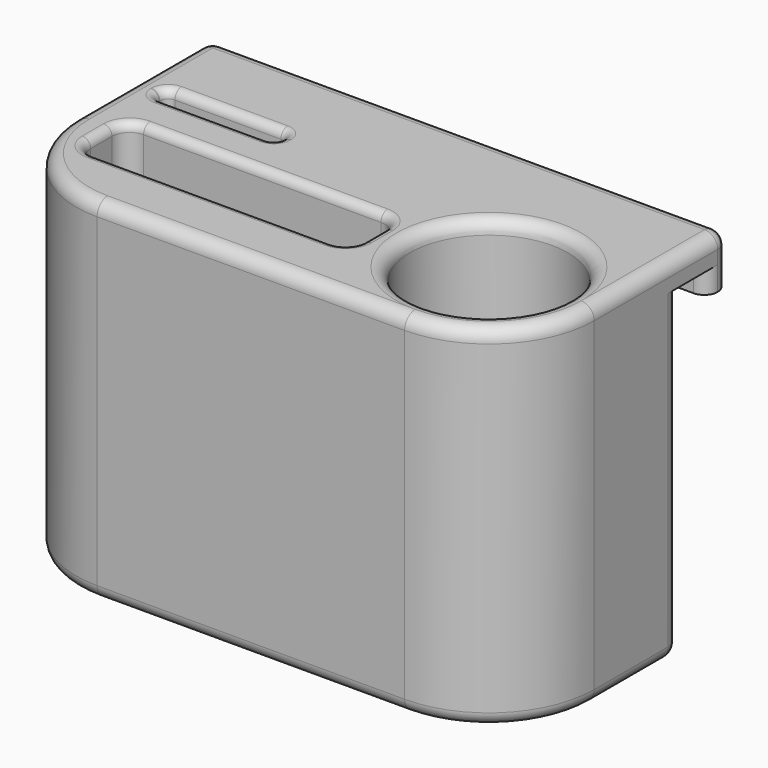
from build123d import *

# Parameters (mm, degrees)
F1_DEPTH     = 93.726
F3_DEPTH     = 63.5
F4_DEPTH     = 60.325
F6_DEPTH     = 63.501
F8_DEPTH     = 60.325
F9_T1_DEPTH  = 88.9508
F9_T3_DEPTH  = 27.9019
F9_T5_DEPTH  = 6.7564
F9_T7_DEPTH  = 56.2864
F9_T9_DEPTH  = 16.7259
F9_T11_DEPTH = 4.318
F9_T13_DEPTH = 55.626
F9_S17_W     = 2.435352
F9_S17_H     = 2.435352
F9_T18_DEPTH = 2.435352
F9_S23_W     = 2.435352
F9_S23_H     = 2.435352
F9_T24_DEPTH = 2.435352
F9_S29_W     = 2.435352
F9_S29_H     = 2.435352
F9_T30_DEPTH = 2.435352
F9_S35_W     = 2.435352
F9_S35_H     = 2.435352
F9_T36_DEPTH = 2.435352
F9_T42_ANGLE = 90
F9_T44_ANGLE = 90
F9_T46_ANGLE = 90
F9_T48_ANGLE = 90
F10_R        = 1.524


# Not quite as in the source:
# - a fillet or chamfer that OpenCascade refuses, or shapes differently, is made with other operations: its cross-section is extruded or revolved along the edge and cut away or added


with BuildPart() as f1:
    # F0 (on Right) → F1 (new body)
    with BuildSketch(Plane.YZ):
        Polygon((-6.35, 0), (0, 0), (0, -4.318), (4.826, -4.318), (4.826, 4.826), (-11.176, 4.826), (-11.176, -58.674), (-6.35, -58.674), align=None)
    extrude(amount=F1_DEPTH)

    # F2 (on face) → F3 (join, through all)
    with BuildSketch(Plane.XY.offset(4.826)):
        with BuildLine():
            Line((93.726, -11.176), (74.676, -11.176))
            Line((74.676, -11.176), (0, -11.176))
            Line((0, -11.176), (0, -25.4635))
            ThreePointArc((0, -25.4635), (5.5796158184, -38.9338841816), (19.05, -44.5135))
            Line((19.05, -44.5135), (74.676, -44.5135))
            ThreePointArc((74.676, -44.5135), (88.1463841816, -38.9338841816), (93.726, -25.4635))
            Line((93.726, -25.4635), (93.726, -11.176))
        make_face()
        with BuildLine():
            ThreePointArc((74.676, -11.176), (84.7787881362, -15.3607118638), (88.9635, -25.4635))
            ThreePointArc((88.9635, -25.4635), (64.5732118638, -35.5662881362), (74.676, -11.176))
        make_face(mode=Mode.SUBTRACT)
        with BuildLine():
            ThreePointArc((74.676, -11.176), (64.5732118638, -35.5662881362), (88.9635, -25.4635))
            ThreePointArc((88.9635, -25.4635), (84.7787881362, -15.3607118638), (74.676, -11.176))
        make_face()
    extrude(amount=-F3_DEPTH)

    # F2 (on face) → F4 (cut)
    with BuildSketch(Plane.XY.offset(4.826)):
        with BuildLine():
            ThreePointArc((74.676, -11.176), (64.5732118638, -35.5662881362), (88.9635, -25.4635))
            ThreePointArc((88.9635, -25.4635), (84.7787881362, -15.3607118638), (74.676, -11.176))
        make_face()
    extrude(amount=-F4_DEPTH, mode=Mode.SUBTRACT)

    # F5 (on face) → F6 (cut, through all)
    with BuildSketch(Plane.XY.offset(4.826)):
        with BuildLine():
            Line((25.527, -11.049), (6.35, -11.049))
            ThreePointArc((6.35, -11.049), (5.2723692655, -11.4953692655), (4.826, -12.573))
            Line((4.826, -12.573), (4.826, -12.7))
            ThreePointArc((4.826, -12.7), (5.2723692655, -13.7776307345), (6.35, -14.224))
            Line((6.35, -14.224), (25.527, -14.224))
            ThreePointArc((25.527, -14.224), (26.6046307345, -13.7776307345), (27.051, -12.7))
            Line((27.051, -12.7), (27.051, -12.573))
            ThreePointArc((27.051, -12.573), (26.6046307345, -11.4953692655), (25.527, -11.049))
        make_face()
    extrude(amount=-F6_DEPTH, mode=Mode.SUBTRACT)

    # F7 (on face) → F8 (cut, through all)
    with BuildSketch(Plane.XY.offset(4.826)):
        with BuildLine():
            ThreePointArc((55.626, -25.273), (54.6960640303, -23.0279359697), (52.451, -22.098))
            Line((52.451, -22.098), (9.525, -22.098))
            ThreePointArc((9.525, -22.098), (7.2799359697, -23.0279359697), (6.35, -25.273))
            Line((6.35, -25.273), (6.35, -30.099))
            ThreePointArc((6.35, -30.099), (7.2799359697, -32.3440640303), (9.525, -33.274))
            Line((9.525, -33.274), (52.451, -33.274))
            ThreePointArc((52.451, -33.274), (54.6960640303, -32.3440640303), (55.626, -30.099))
            Line((55.626, -30.099), (55.626, -25.273))
        make_face()
    extrude(amount=-F8_DEPTH, mode=Mode.SUBTRACT)

    # F9: fillet of radius 2.3876 on 11 edges, made by hand

    # F9_s2 → F9_t1 (cut)
    with BuildSketch(Plane.YZ.offset(2.3876)):
        with BuildLine():
            ThreePointArc((4.826, 2.4384), (4.1266881508, 4.1266881508), (2.4384, 4.826))
            Line((2.4384, 4.826), (2.4384, 4.873752))
            Line((2.4384, 4.873752), (4.873752, 4.873752))
            Line((4.873752, 4.873752), (4.873752, 2.4384))
            Line((4.873752, 2.4384), (4.826, 2.4384))
        make_face()
        with BuildLine():
            ThreePointArc((-8.7376, -58.674), (-7.0493118492, -57.9746881508), (-6.35, -56.2864))
            Line((-6.35, -56.2864), (-6.302248, -56.2864))
            Line((-6.302248, -56.2864), (-6.302248, -58.721752))
            Line((-6.302248, -58.721752), (-8.7376, -58.721752))
            Line((-8.7376, -58.721752), (-8.7376, -58.674))
        make_face()
    extrude(amount=F9_T1_DEPTH, mode=Mode.SUBTRACT)

    # F9_s4 → F9_t3 (cut)
    with BuildSketch(Plane.XZ.offset(-2.4384)):
        with BuildLine():
            ThreePointArc((0, 2.4384), (0.6993118492, 4.1266881508), (2.3876, 4.826))
            Line((2.3876, 4.826), (2.3876, 4.873752))
            Line((2.3876, 4.873752), (-0.047752, 4.873752))
            Line((-0.047752, 4.873752), (-0.047752, 2.4384))
            Line((-0.047752, 2.4384), (0, 2.4384))
        make_face()
        with BuildLine():
            ThreePointArc((93.726, 2.4384), (93.0266881508, 4.1266881508), (91.3384, 4.826))
            Line((91.3384, 4.826), (91.3384, 4.873752))
            Line((91.3384, 4.873752), (93.773752, 4.873752))
            Line((93.773752, 4.873752), (93.773752, 2.4384))
            Line((93.773752, 2.4384), (93.726, 2.4384))
        make_face()
    extrude(amount=F9_T3_DEPTH, mode=Mode.SUBTRACT)

    # F9_s6 → F9_t5 (cut)
    with BuildSketch(Plane.XY.offset(-4.318)):
        with BuildLine():
            ThreePointArc((0, 2.4384), (0.6993118492, 4.1266881508), (2.3876, 4.826))
            Line((2.3876, 4.826), (2.3876, 4.873752))
            Line((2.3876, 4.873752), (-0.047752, 4.873752))
            Line((-0.047752, 4.873752), (-0.047752, 2.4384))
            Line((-0.047752, 2.4384), (0, 2.4384))
        make_face()
        with BuildLine():
            ThreePointArc((93.726, 2.4384), (93.0266881508, 4.1266881508), (91.3384, 4.826))
            Line((91.3384, 4.826), (91.3384, 4.873752))
            Line((91.3384, 4.873752), (93.773752, 4.873752))
            Line((93.773752, 4.873752), (93.773752, 2.4384))
            Line((93.773752, 2.4384), (93.726, 2.4384))
        make_face()
    extrude(amount=F9_T5_DEPTH, mode=Mode.SUBTRACT)

    # F9_s8 → F9_t7 (cut)
    with BuildSketch(Plane.XY.offset(-56.2864)):
        with BuildLine():
            ThreePointArc((2.3876, -6.35), (0.6993118492, -7.0493118492), (0, -8.7376))
            Line((0, -8.7376), (-0.047752, -8.7376))
            Line((-0.047752, -8.7376), (-0.047752, -6.302248))
            Line((-0.047752, -6.302248), (2.3876, -6.302248))
            Line((2.3876, -6.302248), (2.3876, -6.35))
        make_face()
        with BuildLine():
            ThreePointArc((91.3384, -6.35), (93.0266881508, -7.0493118492), (93.726, -8.7376))
            Line((93.726, -8.7376), (93.773752, -8.7376))
            Line((93.773752, -8.7376), (93.773752, -6.302248))
            Line((93.773752, -6.302248), (91.3384, -6.302248))
            Line((91.3384, -6.302248), (91.3384, -6.35))
        make_face()
    extrude(amount=F9_T7_DEPTH, mode=Mode.SUBTRACT)

    # F9_s10 → F9_t9 (cut)
    with BuildSketch(Plane.XZ.offset(8.7376)):
        with BuildLine():
            ThreePointArc((2.3876, -58.674), (0.6993118492, -57.9746881508), (0, -56.2864))
            Line((0, -56.2864), (-0.047752, -56.2864))
            Line((-0.047752, -56.2864), (-0.047752, -58.721752))
            Line((-0.047752, -58.721752), (2.3876, -58.721752))
            Line((2.3876, -58.721752), (2.3876, -58.674))
        make_face()
        with BuildLine():
            ThreePointArc((91.3384, -58.674), (93.0266881508, -57.9746881508), (93.726, -56.2864))
            Line((93.726, -56.2864), (93.773752, -56.2864))
            Line((93.773752, -56.2864), (93.773752, -58.721752))
            Line((93.773752, -58.721752), (91.3384, -58.721752))
            Line((91.3384, -58.721752), (91.3384, -58.674))
        make_face()
    extrude(amount=F9_T9_DEPTH, mode=Mode.SUBTRACT)

    # F9_s12 → F9_t11 (cut)
    with BuildSketch(Plane.XY.offset(-4.318)):
        with BuildLine():
            ThreePointArc((0, 2.3876), (0.6993118492, 0.6993118492), (2.3876, 0))
            Line((2.3876, 0), (2.3876, -0.047752))
            Line((2.3876, -0.047752), (-0.047752, -0.047752))
            Line((-0.047752, -0.047752), (-0.047752, 2.3876))
            Line((-0.047752, 2.3876), (0, 2.3876))
        make_face()
        with BuildLine():
            ThreePointArc((93.726, 2.3876), (93.0266881508, 0.6993118492), (91.3384, 0))
            Line((91.3384, 0), (91.3384, -0.047752))
            Line((91.3384, -0.047752), (93.773752, -0.047752))
            Line((93.773752, -0.047752), (93.773752, 2.3876))
            Line((93.773752, 2.3876), (93.726, 2.3876))
        make_face()
    extrude(amount=F9_T11_DEPTH, mode=Mode.SUBTRACT)

    # F9_s14 → F9_t13 (cut)
    with BuildSketch(Plane.YZ.offset(19.05)):
        with BuildLine():
            ThreePointArc((-42.1259, -58.674), (-43.8141881508, -57.9746881508), (-44.5135, -56.2864))
            Line((-44.5135, -56.2864), (-44.561252, -56.2864))
            Line((-44.561252, -56.2864), (-44.561252, -58.721752))
            Line((-44.561252, -58.721752), (-42.1259, -58.721752))
            Line((-42.1259, -58.721752), (-42.1259, -58.674))
        make_face()
        with BuildLine():
            ThreePointArc((-44.5135, 2.4384), (-43.8141881508, 4.1266881508), (-42.1259, 4.826))
            Line((-42.1259, 4.826), (-42.1259, 4.873752))
            Line((-42.1259, 4.873752), (-44.561252, 4.873752))
            Line((-44.561252, 4.873752), (-44.561252, 2.4384))
            Line((-44.561252, 2.4384), (-44.5135, 2.4384))
        make_face()
    extrude(amount=F9_T13_DEPTH, mode=Mode.SUBTRACT)


with BuildPart() as f9_tool16:
    # F9_s17 → F9_t18 (new body)
    with BuildSketch(Plane.YZ.offset(2.3876)):
        with Locations((3.656076, 3.656076)):
            Rectangle(F9_S17_W, F9_S17_H)
    extrude(amount=-F9_T18_DEPTH)

    # F9_s19 → F9_t20 (revolve, cut)
    with BuildSketch(Plane(origin=(2.3876, 2.4384, 2.4384), x_dir=(0, -0.7071067812, -0.7071067812), z_dir=(0, 0.7071067812, -0.7071067812))):
        with BuildLine():
            ThreePointArc((0, -2.3876), (2.3876, 0), (0, 2.3876))
            Line((0, 2.3876), (0, -2.3876))
        make_face()
    revolve(axis=Axis((2.3876, 2.4384, 2.4384), (-1, 0, 0)), mode=Mode.SUBTRACT)


with BuildPart() as f1_1:
    add(f1.part)

    # F9_t15: cut F9_tool16
    add(f9_tool16.part, mode=Mode.SUBTRACT)


with BuildPart() as f9_tool22:
    # F9_s23 → F9_t24 (new body)
    with BuildSketch(Plane.YZ.offset(91.3384)):
        with Locations((3.656076, 3.656076)):
            Rectangle(F9_S23_W, F9_S23_H)
    extrude(amount=F9_T24_DEPTH)

    # F9_s25 → F9_t26 (revolve, cut)
    with BuildSketch(Plane(origin=(91.3384, 2.4384, 2.4384), x_dir=(0, -0.7071067812, -0.7071067812), z_dir=(0, -0.7071067812, 0.7071067812))):
        with BuildLine():
            ThreePointArc((0, -2.3876), (2.3876, 0), (0, 2.3876))
            Line((0, 2.3876), (0, -2.3876))
        make_face()
    revolve(axis=Axis((91.3384, 2.4384, 2.4384), (1, 0, 0)), mode=Mode.SUBTRACT)


with BuildPart() as f1_2:
    add(f1_1.part)

    # F9_t21: cut F9_tool22
    add(f9_tool22.part, mode=Mode.SUBTRACT)


with BuildPart() as f9_tool28:
    # F9_s29 → F9_t30 (new body)
    with BuildSketch(Plane.XY.offset(-56.2864)):
        with Locations((1.169924, -7.519924)):
            Rectangle(F9_S29_W, F9_S29_H)
    extrude(amount=-F9_T30_DEPTH)

    # F9_s31 → F9_t32 (revolve, cut)
    with BuildSketch(Plane(origin=(2.3876, -8.7376, -56.2864), x_dir=(0.7071067812, -0.7071067812, 0), z_dir=(0.7071067812, 0.7071067812, 0))):
        with BuildLine():
            ThreePointArc((0, -2.3876), (2.3876, 0), (0, 2.3876))
            Line((0, 2.3876), (0, -2.3876))
        make_face()
    revolve(axis=Axis((2.3876, -8.7376, -56.2864), (0, 0, -1)), mode=Mode.SUBTRACT)


with BuildPart() as f1_3:
    add(f1_2.part)

    # F9_t27: cut F9_tool28
    add(f9_tool28.part, mode=Mode.SUBTRACT)


with BuildPart() as f9_tool34:
    # F9_s35 → F9_t36 (new body)
    with BuildSketch(Plane.XY.offset(-56.2864)):
        with Locations((92.556076, -7.519924)):
            Rectangle(F9_S35_W, F9_S35_H)
    extrude(amount=-F9_T36_DEPTH)

    # F9_s37 → F9_t38 (revolve, cut)
    with BuildSketch(Plane(origin=(91.3384, -8.7376, -56.2864), x_dir=(-0.7071067812, -0.7071067812, 0), z_dir=(0.7071067812, -0.7071067812, 0))):
        with BuildLine():
            ThreePointArc((0, -2.3876), (2.3876, 0), (0, 2.3876))
            Line((0, 2.3876), (0, -2.3876))
        make_face()
    revolve(axis=Axis((91.3384, -8.7376, -56.2864), (0, 0, -1)), mode=Mode.SUBTRACT)


with BuildPart() as f1_4:
    add(f1_3.part)

    # F9_t33: cut F9_tool34
    add(f9_tool34.part, mode=Mode.SUBTRACT)

    # F9_s39 → F9_t40 (revolve, cut)
    with BuildSketch(Plane.XZ.offset(25.4635)):
        with BuildLine():
            ThreePointArc((91.3511, 4.826), (89.6628118492, 4.1266881508), (88.9635, 2.4384))
            Line((88.9635, 2.4384), (88.915748, 2.4384))
            Line((88.915748, 2.4384), (88.915748, 4.873752))
            Line((88.915748, 4.873752), (91.3511, 4.873752))
            Line((91.3511, 4.873752), (91.3511, 4.826))
        make_face()
    revolve(axis=Axis((74.676, -25.4635, 4.826), (0, 0, -1)), mode=Mode.SUBTRACT)

    # F9_s41 → F9_t42 (revolve, cut)
    with BuildSketch(Plane.XZ.offset(25.4635)):
        with BuildLine():
            ThreePointArc((2.3876, -58.674), (0.6993118492, -57.9746881508), (0, -56.2864))
            Line((0, -56.2864), (-0.047752, -56.2864))
            Line((-0.047752, -56.2864), (-0.047752, -58.721752))
            Line((-0.047752, -58.721752), (2.3876, -58.721752))
            Line((2.3876, -58.721752), (2.3876, -58.674))
        make_face()
    revolve(axis=Axis((19.05, -25.4635, -58.674), (0, 0, 1)), revolution_arc=F9_T42_ANGLE, mode=Mode.SUBTRACT)

    # F9_s43 → F9_t44 (revolve, cut)
    with BuildSketch(Plane.YZ.offset(74.676)):
        with BuildLine():
            ThreePointArc((-42.1259, -58.674), (-43.8141881508, -57.9746881508), (-44.5135, -56.2864))
            Line((-44.5135, -56.2864), (-44.561252, -56.2864))
            Line((-44.561252, -56.2864), (-44.561252, -58.721752))
            Line((-44.561252, -58.721752), (-42.1259, -58.721752))
            Line((-42.1259, -58.721752), (-42.1259, -58.674))
        make_face()
    revolve(axis=Axis((74.676, -25.4635, -58.674), (0, 0, 1)), revolution_arc=F9_T44_ANGLE, mode=Mode.SUBTRACT)

    # F9_s45 → F9_t46 (revolve, cut)
    with BuildSketch(Plane.XZ.offset(25.4635)):
        with BuildLine():
            ThreePointArc((0, 2.4384), (0.6993118492, 4.1266881508), (2.3876, 4.826))
            Line((2.3876, 4.826), (2.3876, 4.873752))
            Line((2.3876, 4.873752), (-0.047752, 4.873752))
            Line((-0.047752, 4.873752), (-0.047752, 2.4384))
            Line((-0.047752, 2.4384), (0, 2.4384))
        make_face()
    revolve(axis=Axis((19.05, -25.4635, 4.826), (0, 0, 1)), revolution_arc=F9_T46_ANGLE, mode=Mode.SUBTRACT)

    # F9_s47 → F9_t48 (revolve, cut)
    with BuildSketch(Plane.YZ.offset(74.676)):
        with BuildLine():
            ThreePointArc((-44.5135, 2.4384), (-43.8141881508, 4.1266881508), (-42.1259, 4.826))
            Line((-42.1259, 4.826), (-42.1259, 4.873752))
            Line((-42.1259, 4.873752), (-44.561252, 4.873752))
            Line((-44.561252, 4.873752), (-44.561252, 2.4384))
            Line((-44.561252, 2.4384), (-44.5135, 2.4384))
        make_face()
    revolve(axis=Axis((74.676, -25.4635, 4.826), (0, 0, 1)), revolution_arc=F9_T48_ANGLE, mode=Mode.SUBTRACT)

    # F10
    f10_edges = [f1_4.edges().sort_by_distance(p)[0] for p in [
        (15.9385, -11.049, 4.826),
        (26.604631, -13.777631, -58.674),
        (30.988, -22.098, 4.826),
        (30.988, -33.274, -55.499),
        (60.3885, -25.4635, -55.499),
    ]]
    fillet(f10_edges, radius=F10_R)


solid = f1_4.part
